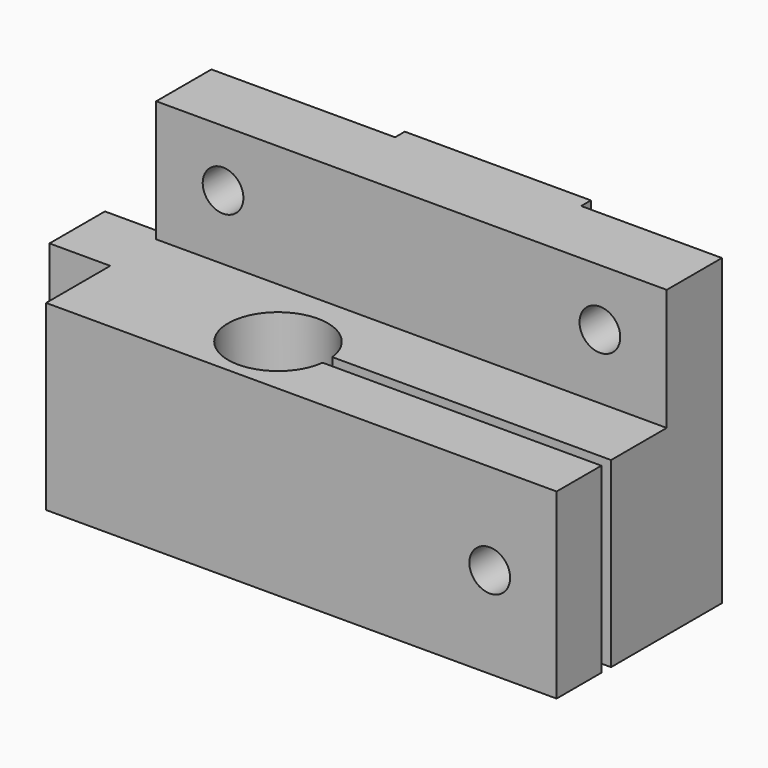
from build123d import *

# Parameters (mm, degrees)
F0_W          = 42
F0_H          = 17
F1_DEPTH      = 15
F3_R          = 1.675
F4_DEPTH      = 16
F5_W          = 42
F5_H          = 5.6745335534
F6_DEPTH      = 10
F7_R          = 1.675
F8_DEPTH      = 25
F9_DEPTH      = 25
F10_TEXT_SIZE = 34.7222222222
F11_DEPTH     = 1
F12_W         = 5.7
F12_H         = 15
F13_DEPTH     = 5


# Not quite as in the source:
# - Text() gives the source's letters only with a copy of the font that has no kerning and outlines rounded to 1/6400 em; it was checked with that copy


with BuildPart() as f1:
    # F0 (on Top) → F1 (new body)
    with BuildSketch(Plane.XY):
        with Locations((21, 8.5)):
            Rectangle(F0_W, F0_H)
    extrude(amount=F1_DEPTH)

    # F3 (on face) → F4 (cut)
    with BuildSketch(Plane.XZ):
        with Locations((36.5, 7.5)):
            Circle(F3_R)
    extrude(amount=-F4_DEPTH, mode=Mode.SUBTRACT)

    # F5 (on face) → F6 (join)
    with BuildSketch(Plane.XY.offset(15)):
        with Locations((21, 14.1627332233)):
            Rectangle(F5_W, F5_H)
    extrude(amount=F6_DEPTH)

    # F7 (on face) → F8 (cut)
    with BuildSketch(Plane(origin=(0, 17, 0), x_dir=(-1, 0, 0), z_dir=(0, 1, 0))):
        with Locations((-36.5, 20.325)):
            Circle(F7_R)
        with Locations((-5.5, 20.325)):
            Circle(F7_R)
    extrude(amount=-F8_DEPTH, mode=Mode.SUBTRACT)

    # F2 (on face) → F9 (cut)
    with BuildSketch(Plane.XY.offset(15)):
        with BuildLine():
            ThreePointArc((19.0693979899, 4.6), (19.0923423463, 4.8495321962), (19.1, 5.1))
            ThreePointArc((19.1, 5.1), (19.0923423463, 5.3504678038), (19.0693979899, 5.6))
            ThreePointArc((19.0693979899, 5.6), (10.9, 5.1), (19.0693979899, 4.6))
        make_face()
        with BuildLine():
            Line((42, 5.1), (19.1, 5.1))
            ThreePointArc((19.1, 5.1), (19.0923423463, 4.8495321962), (19.0693979899, 4.6))
            Line((19.0693979899, 4.6), (42, 4.6))
            Line((42, 4.6), (42, 5.1))
        make_face()
        with BuildLine():
            ThreePointArc((19.0693979899, 5.6), (19.0923423463, 5.3504678038), (19.1, 5.1))
            Line((19.1, 5.1), (42, 5.1))
            Line((42, 5.1), (42, 5.6))
            Line((42, 5.6), (19.0693979899, 5.6))
        make_face()
    extrude(amount=-F9_DEPTH, mode=Mode.SUBTRACT)

    # F10 (on face) → F11 (join)
    with BuildSketch(Plane(origin=(0, 17, 0), x_dir=(-1, 0, 0), z_dir=(0, 1, 0))):
        with Locations(Location((-11.9905544113, 25), (0, 0, 180))):
            Text('L', F10_TEXT_SIZE, font='Open Sans', font_style=FontStyle.BOLD, text_align=(TextAlign.LEFT, TextAlign.BOTTOM))
    extrude(amount=F11_DEPTH)

    # F12 (on face) → F13 (join)
    with BuildSketch(Plane(origin=(0, 0, 0), x_dir=(0, -1, 0), z_dir=(-1, 0, 0))):
        with Locations((-9.45, 7.5)):
            Rectangle(F12_W, F12_H)
    extrude(amount=F13_DEPTH)


solid = f1.part
